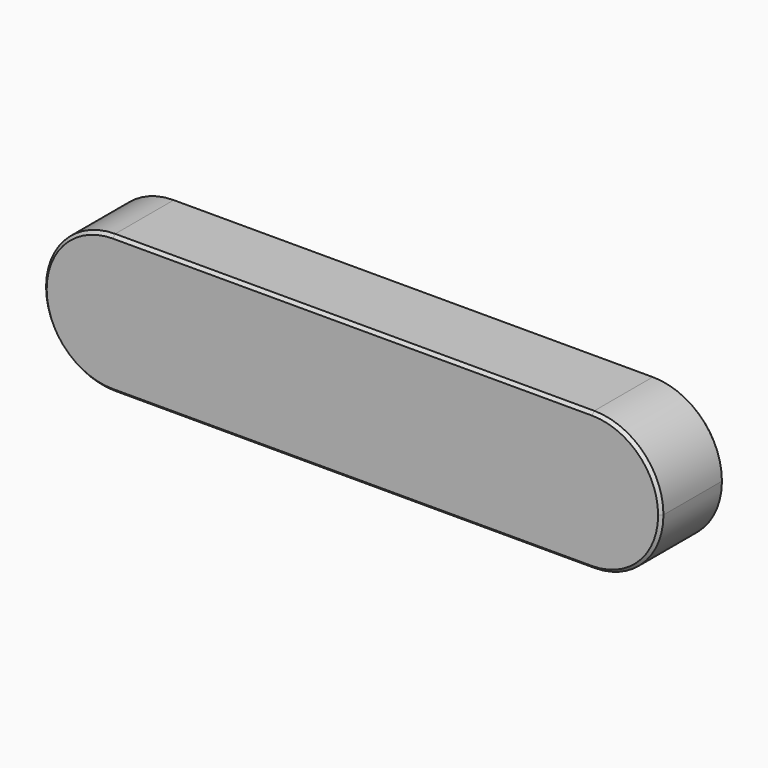
from build123d import *

# Parameters (mm, degrees)
F0_W     = 125
F0_H     = 28
F1_DEPTH = 8
F2_R     = 13.99999
F3_SIZE  = 0.6


# Not quite as in the source:
# - a fillet or chamfer is up to 0.001 mm smaller than in the source, because OpenCascade refuses the exact size


with BuildPart() as f1:
    # F0 (on Front) → F1 (new body, symmetric)
    with BuildSketch(Plane.XZ):
        Rectangle(F0_W, F0_H)
    extrude(amount=F1_DEPTH, both=True)

    # F2 (radius 14 in the source; OpenCascade refuses exactly that, so slightly less here)
    f2_edges = [f1.edges().sort_by_distance(p)[0] for p in [
        (62.5, 0, -14),
        (62.5, 0, 14),
        (-62.5, 0, -14),
        (-62.5, 0, 14),
    ]]
    fillet(f2_edges, radius=F2_R)

    # F3
    f3_edges = [f1.edges().sort_by_distance(p)[0] for p in [
        (0, -8, 14),
        (62.5, -8, 0),
        (58.399498, -8, -9.899498),
        (58.399498, -8, 9.899498),
        (0, -8, -14),
        (-58.399498, -8, -9.899498),
        (-58.399498, -8, 9.899498),
        (-62.5, -8, 0),
        (62.5, 8, 0),
        (58.399498, 8, -9.899498),
        (58.399498, 8, 9.899498),
        (0, 8, -14),
        (0, 8, 14),
        (-58.399498, 8, -9.899498),
        (-58.399498, 8, 9.899498),
        (-62.5, 8, 0),
    ]]
    chamfer(f3_edges, length=F3_SIZE)


solid = f1.part
